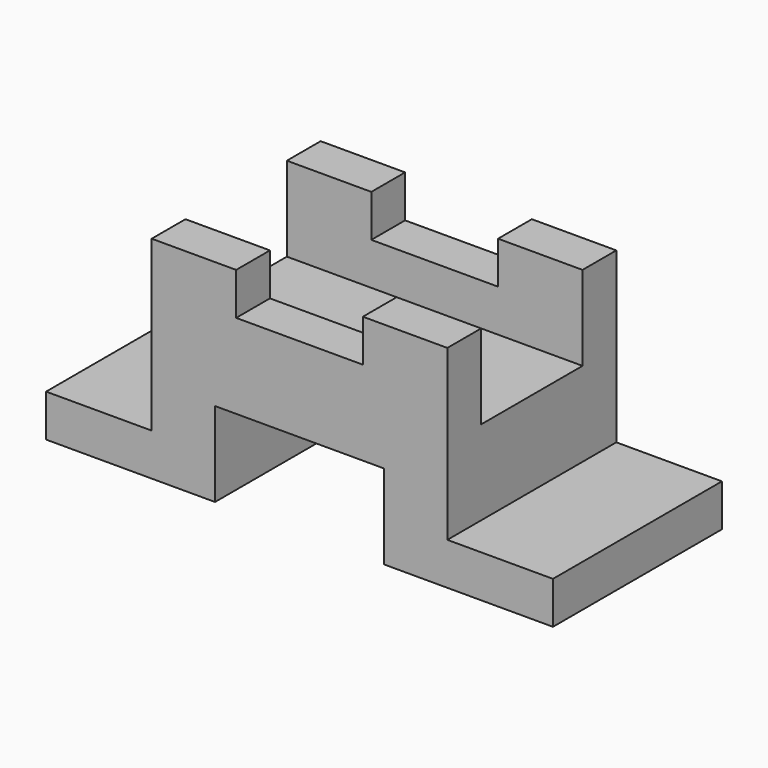
from build123d import *

# Parameters (mm, degrees)
F1_W     = 1016
F1_H     = 508
F2_DEPTH = 1270
F3_DEPTH = 1270.001
F4_W     = 508
F4_H     = 762
F5_DEPTH = 508
F6_W     = 508
F6_H     = 762
F7_DEPTH = 508
F8_W     = 762
F8_H     = 762
F9_DEPTH = 254


# Not quite as in the source:
# - a variable given as a bare number and used for a length is read in inches; the dataset says mm whatever the document's units were


with BuildPart() as f2:
    # F1 (on Front) → F2 (new body)
    with BuildSketch(Plane.XZ):
        Polygon((-1450.5924028924, 254), (-1450.5924028924, 0), (-434.5924028924, 0), (-434.5924028924, 508), (581.4075971076, 508), (581.4075971076, 0), (1597.4075971076, 0), (1597.4075971076, 254), (962.4075971076, 254), (962.4075971076, 1270), (454.4075971076, 1270), (454.4075971076, 1016), (-307.5924028924, 1016), (-307.5924028924, 1270), (-815.5924028924, 1270), (-815.5924028924, 254), align=None)
        with Locations((73.4075971076, 254)):
            Rectangle(F1_W, F1_H)
    extrude(amount=-F2_DEPTH)

    # F1 (on Front) → F3 (cut, through all)
    with BuildSketch(Plane.XZ):
        with Locations((73.4075971076, 254)):
            Rectangle(F1_W, F1_H)
    extrude(amount=-F3_DEPTH, mode=Mode.SUBTRACT)

    # F4 (on face) → F5 (cut)
    with BuildSketch(Plane.XY.offset(1270)):
        with Locations((-561.5924028924, 635)):
            Rectangle(F4_W, F4_H)
    extrude(amount=-F5_DEPTH, mode=Mode.SUBTRACT)

    # F6 (on face) → F7 (cut)
    with BuildSketch(Plane.XY.offset(1270)):
        with Locations((708.4075971076, 635)):
            Rectangle(F6_W, F6_H)
    extrude(amount=-F7_DEPTH, mode=Mode.SUBTRACT)

    # F8 (on face) → F9 (cut)
    with BuildSketch(Plane.XY.offset(1016)):
        with Locations((73.4075971076, 635)):
            Rectangle(F8_W, F8_H)
    extrude(amount=-F9_DEPTH, mode=Mode.SUBTRACT)


solid = f2.part
